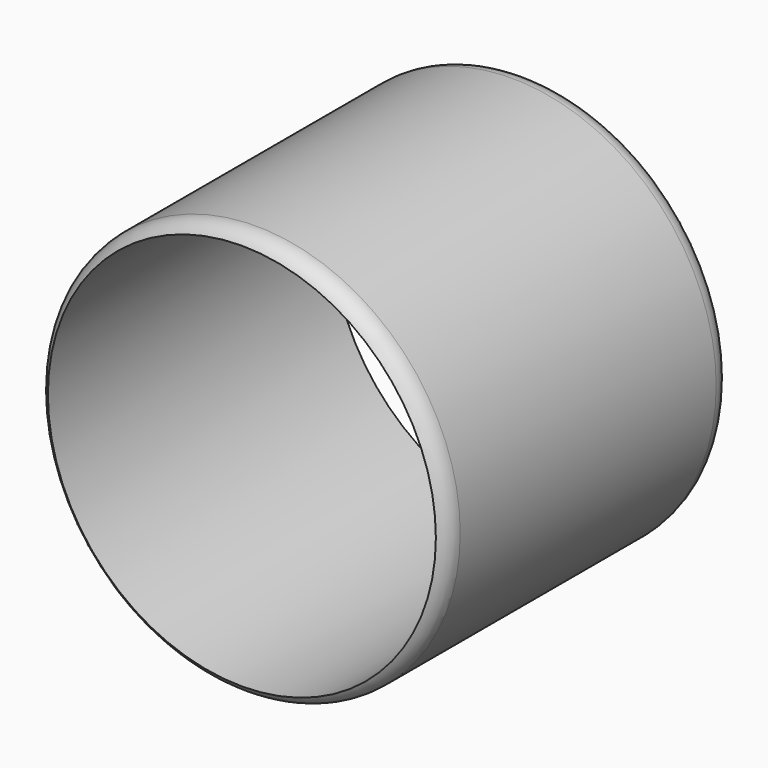
from build123d import *

# Parameters (mm, degrees)
F0_R     = 50
F1_DEPTH = 87
F3_D     = 95
F3_DEPTH = 100
F3_TIP   = 28.5408794038


# Not quite as in the source:
# - a fillet or chamfer that OpenCascade refuses, or shapes differently, is made with other operations: its cross-section is extruded or revolved along the edge and cut away or added


with BuildPart() as f1:
    # F0 (on Front) → F1 (new body)
    with BuildSketch(Plane.XZ):
        Circle(F0_R)
    extrude(amount=-F1_DEPTH)

    # F3
    with Locations(Plane.XZ):
        with Locations((0, 0)):
            Hole(F3_D / 2, depth=F3_DEPTH)
            with Locations((0, 0, -(F3_DEPTH + F3_TIP / 2))):  # 118° drill point
                Cone(0, F3_D / 2, F3_TIP, mode=Mode.SUBTRACT)

    # F4: fillet of radius 5 on 2 edges, made by hand

    # F4_s1 → F4_t2 (revolve, cut)
    with BuildSketch(Plane.XY):
        with BuildLine():
            ThreePointArc((50, 4.3301270189), (49.3301270189, 1.8301270189), (47.5, 0))
            Line((47.5, 0), (50, 0))
            Line((50, 0), (50, 4.3301270189))
        make_face()
    revolve(axis=Axis((0, 0, 0), (0, -1, 0)), mode=Mode.SUBTRACT)

    # F4_s3 → F4_t4 (revolve, cut)
    with BuildSketch(Plane.XY):
        with BuildLine():
            ThreePointArc((50, 82.6698729811), (49.3301270189, 85.1698729811), (47.5, 87))
            Line((47.5, 87), (50, 87))
            Line((50, 87), (50, 82.6698729811))
        make_face()
    revolve(axis=Axis((0, 87, 0), (0, -1, 0)), mode=Mode.SUBTRACT)


solid = f1.part
